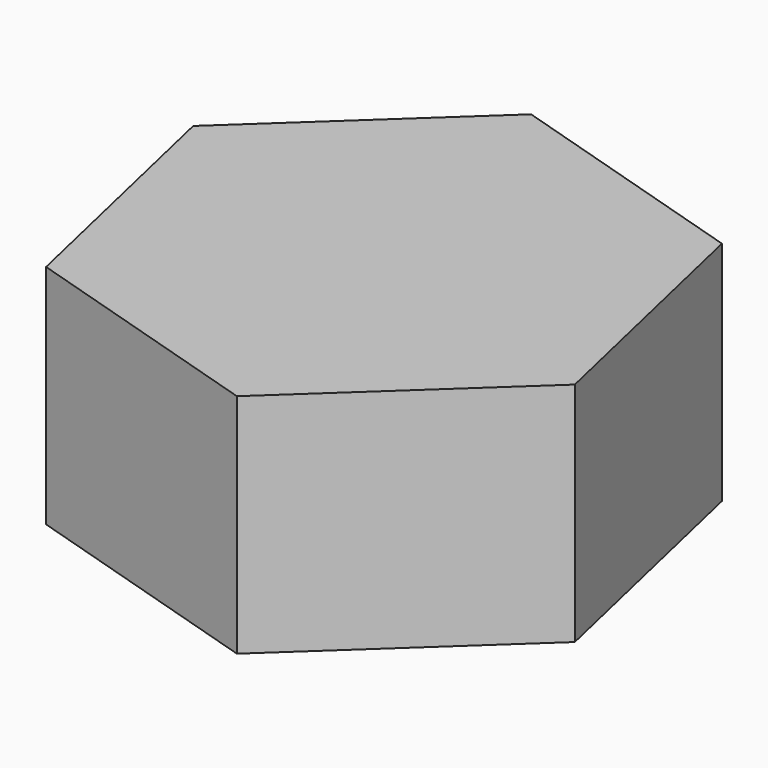
from build123d import *

# Parameters (mm, degrees)
F1_DEPTH = 5.5


# Not quite as in the source:
# - a feature names something its author has since deleted; it is built from what else it names


with BuildPart() as f1:
    # F0 (on Top) → F1 (new body)
    with BuildSketch(Plane.XY):
        Polygon((1.4364314693, -6.2573794808), (6.1372653262, -1.8847035972), (4.7008338569, 4.3726758837), (-1.4364314693, 6.2573794808), (-6.1372653262, 1.8847035972), (-4.7008338569, -4.3726758837), align=None)
    extrude(amount=F1_DEPTH)


solid = f1.part
